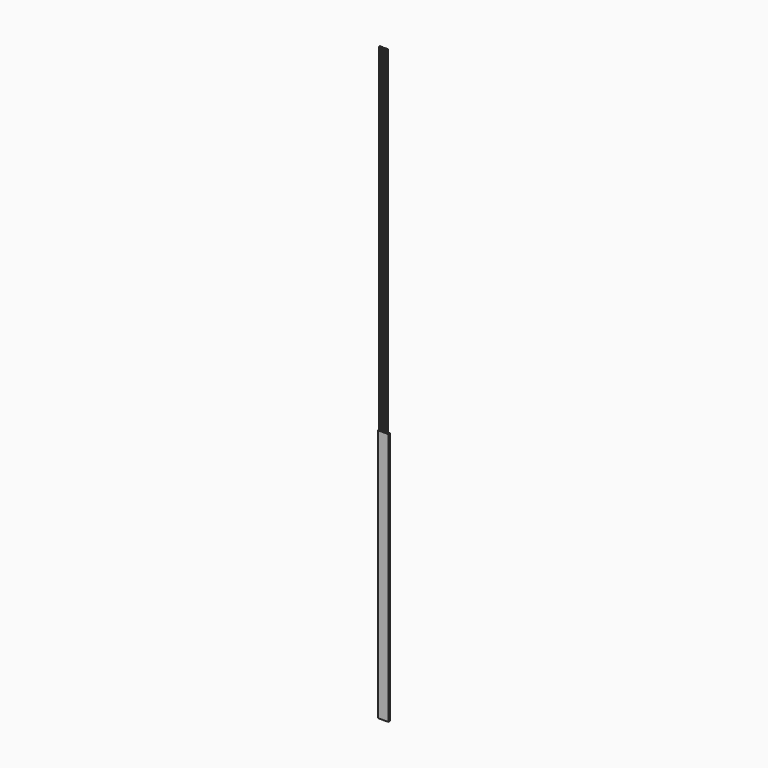
from build123d import *

# Parameters (mm, degrees)
F1_W         = 121.6797716916
F1_H         = 26.2327883393
F1_R         = 3.080204427
F2_DEPTH     = 3000
F0_TEXT_SIZE = 18.7124746541
F3_DEPTH     = 7000


# Not quite as in the source:
# - Text() gives the source's letters only with a copy of the font that has no kerning and outlines rounded to 1/6400 em; it was checked with that copy


with BuildPart() as f2:
    # F1 (on Top) → F2 (new body)
    with BuildSketch(Plane.XY):
        with Locations((26.3336803764, 40.862611495)):
            Rectangle(F1_W, F1_H)
        with Locations((82.1288004518, 48.9342398942)):
            Circle(F1_R, mode=Mode.SUBTRACT)
    extrude(amount=F2_DEPTH)

    # F0 (on Top) → F3 (join)
    with BuildSketch(Plane.XY):
        with Locations((-28.7385396659, 34.9114984274)):
            Text('Makerfaire', F0_TEXT_SIZE, font='Open Sans', font_style=FontStyle.BOLDITALIC, text_align=(TextAlign.LEFT, TextAlign.BOTTOM))
    extrude(amount=F3_DEPTH)


solid = f2.part
